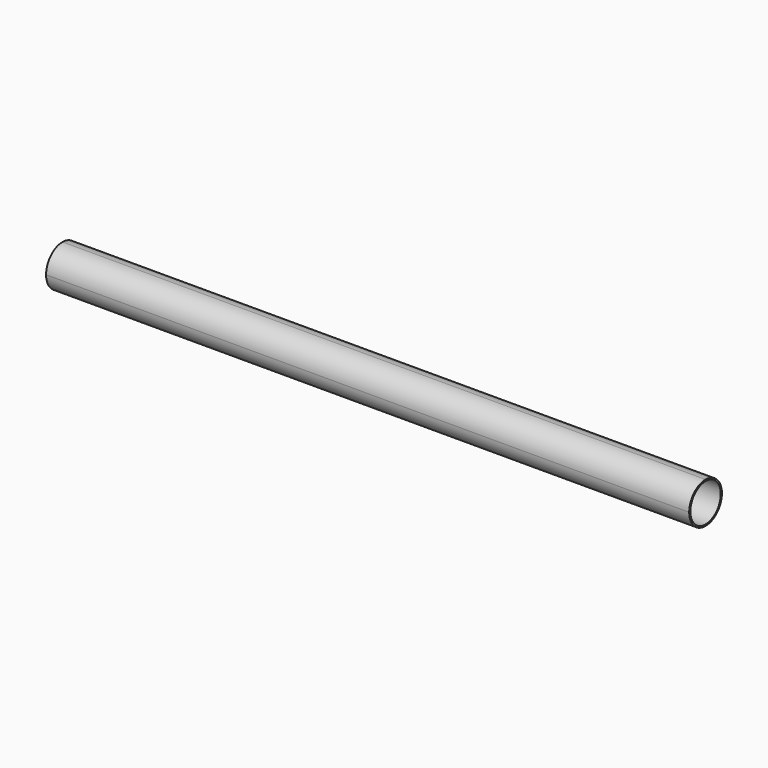
from build123d import *

# Parameters (mm, degrees)
F0_W     = 110
F0_H     = 7
F1_DEPTH = 7
F3_R     = 3.49999
F6_D     = 6.5
F6_DEPTH = 40
F6_TIP   = 1.9527970118
F7_D     = 6.5
F7_DEPTH = 40
F7_TIP   = 1.9527970118


# Not quite as in the source:
# - a fillet or chamfer is up to 0.001 mm smaller than in the source, because OpenCascade refuses the exact size


with BuildPart() as f1:
    # F0 (on Top) → F1 (new body)
    with BuildSketch(Plane.XY):
        Rectangle(F0_W, F0_H)
    extrude(amount=F1_DEPTH)

    # F3 (radius 3.5 in the source; OpenCascade refuses exactly that, so slightly less here)
    f3_edges = [f1.edges().sort_by_distance(p)[0] for p in [
        (0, -3.5, 7),
        (0, 3.5, 7),
        (0, 3.5, 0),
        (0, -3.5, 0),
    ]]
    fillet(f3_edges, radius=F3_R)

    # F6
    with Locations(Plane.YZ.offset(55)):
        with Locations((0, 3.5)):
            Hole(F6_D / 2, depth=F6_DEPTH)
            with Locations((0, 0, -(F6_DEPTH + F6_TIP / 2))):  # 118° drill point
                Cone(0, F6_D / 2, F6_TIP, mode=Mode.SUBTRACT)

    # F7
    with Locations(Plane(origin=(-55, 0, 0), x_dir=(0, -1, 0), z_dir=(-1, 0, 0))):
        with Locations((0, 3.4602470696)):
            Hole(F7_D / 2, depth=F7_DEPTH)
            with Locations((0, 0, -(F7_DEPTH + F7_TIP / 2))):  # 118° drill point
                Cone(0, F7_D / 2, F7_TIP, mode=Mode.SUBTRACT)


solid = f1.part
